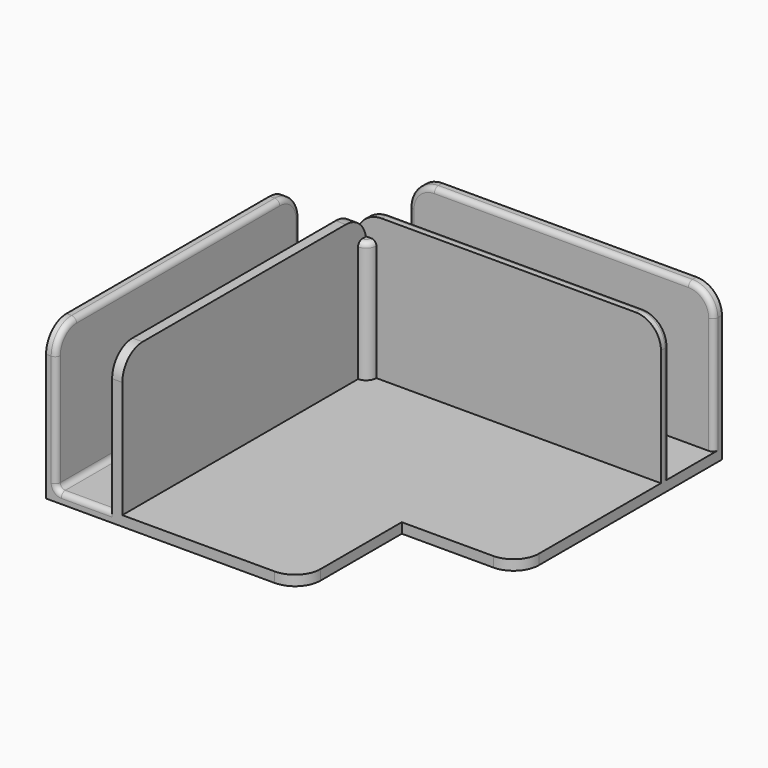
from build123d import *

# Parameters (mm, degrees)
F0_W         = 2
F0_H         = 2
F0_W_2       = 11
F0_H_2       = 28
F0_W_3       = 35
F1_DEPTH     = 60
F2_ANGLE     = -90
F4_R         = 5
F4_2_R       = 5
F6_DEPTH     = 23.9
F7_R         = 1.99999
F8_T1_DEPTH  = 60
F8_T3_DEPTH  = 23
F8_T5_DEPTH  = 1e-05
F8_T7_DEPTH  = 1e-05
F8_T9_DEPTH  = 50
F8_T12_ANGLE = 90
F8_T14_ANGLE = 90
F8_T16_ANGLE = 90
F8_T18_ANGLE = 90
F8_T20_ANGLE = 90
F8_T21_DEPTH = 50
F8_T23_DEPTH = 22
F8_T25_DEPTH = 10
F8_T28_ANGLE = 90
F8_T30_ANGLE = 90
F8_T32_ANGLE = 90
F8_T34_ANGLE = 90


# Not quite as in the source:
# - a fillet or chamfer that OpenCascade refuses, or shapes differently, is made with other operations: its cross-section is extruded or revolved along the edge and cut away or added
# - a fillet or chamfer is up to 0.001 mm smaller than in the source, because OpenCascade refuses the exact size


with BuildPart() as f1:
    # F0 (on Front) → F1 (new body)
    with BuildSketch(Plane.XZ):
        with Locations((1, 1)):
            Rectangle(F0_W, F0_H)
        with Locations((7.5, 1)):
            Rectangle(F0_W_2, F0_H)
        with Locations((1, 16)):
            Rectangle(F0_W, F0_H_2)
        with Locations((14, 1)):
            Rectangle(F0_W, F0_H)
        with Locations((32.5, 1)):
            Rectangle(F0_W_3, F0_H)
        with Locations((14, 16)):
            Rectangle(F0_W, F0_H_2)
    extrude(amount=F1_DEPTH)


with BuildPart() as f2_1:
    # F2: copy of F1
    add(f1.part.rotate(Axis((15, 0, 16), (0, 0, 1)), F2_ANGLE))


with BuildPart() as f2_1_1:
    # F3: moved
    add(f2_1.part.moved(Location((58, 0, 0))))

    # F4#2
    f4_2_edges = [f2_1_1.edges().sort_by_distance(p)[0] for p in [
        (73, 1, 30),
        (73, 14, 30),
        (13, 14, 30),
        (13, 1, 30),
        (73, -35, 1),
    ]]
    fillet(f4_2_edges, radius=F4_2_R)


with BuildPart() as f1_1:
    add(f1.part)

    # F4
    f4_edges = [f1_1.edges().sort_by_distance(p)[0] for p in [
        (14, 0, 30),
        (1, 0, 30),
        (14, -60, 30),
        (1, -60, 30),
        (50, -60, 1),
    ]]
    fillet(f4_edges, radius=F4_R)

    add(f2_1_1.part)  # F6 merges F2_1
    # F5 (on face) → F6 (join)
    with BuildSketch(Plane.XY.offset(2)):
        Polygon((16.8020091951, 0), (15, 0), (15, -2), (17, -2), (17, 0), align=None)
    extrude(amount=F6_DEPTH)

    # F7 (radius 2 in the source; OpenCascade refuses exactly that, so slightly less here)
    f7_edges = [f1_1.edges().sort_by_distance(p)[0] for p in [
        (17, -2, 13.95),
    ]]
    fillet(f7_edges, radius=F7_R)

    # F8: fillet of radius 1 on 19 edges, made by hand

    # F8_s2 → F8_t1 (join)
    with BuildSketch(Plane.XZ):
        with BuildLine():
            ThreePointArc((2, 3), (2.2928932188, 2.2928932188), (3, 2))
            Line((3, 2), (2, 2))
            Line((2, 2), (2, 3))
        make_face()
    extrude(amount=F8_T1_DEPTH)

    # F8_s4 → F8_t3 (cut)
    with BuildSketch(Plane.XY.offset(2)):
        with BuildLine():
            ThreePointArc((13, 1), (13.2928932188, 1.7071067812), (14, 2))
            Line((14, 2), (13, 2))
            Line((13, 2), (13, 1))
        make_face()
        with BuildLine():
            ThreePointArc((73, 14), (72.7071067812, 13.2928932188), (72, 13))
            Line((72, 13), (73, 13))
            Line((73, 13), (73, 14))
        make_face()
        with BuildLine():
            ThreePointArc((73, 1), (72.7071067812, 1.7071067812), (72, 2))
            Line((72, 2), (73, 2))
            Line((73, 2), (73, 1))
        make_face()
        with BuildLine():
            ThreePointArc((13, 14), (13.2928932188, 13.2928932188), (14, 13))
            Line((14, 13), (13, 13))
            Line((13, 13), (13, 14))
        make_face()
    extrude(amount=F8_T3_DEPTH, mode=Mode.SUBTRACT)

    # F8_s6 → F8_t5 (cut)
    with BuildSketch(Plane.YZ.offset(15)):
        with BuildLine():
            ThreePointArc((-2, 24.9), (-1.7071067812, 25.6071067812), (-1, 25.9))
            Line((-1, 25.9), (-2, 25.9))
            Line((-2, 25.9), (-2, 24.9))
        make_face()
    extrude(amount=F8_T5_DEPTH, mode=Mode.SUBTRACT)

    # F8_s8 → F8_t7 (cut)
    with BuildSketch(Plane.XZ):
        with BuildLine():
            ThreePointArc((17, 24.9), (16.7071067812, 25.6071067812), (16, 25.9))
            Line((16, 25.9), (17, 25.9))
            Line((17, 25.9), (17, 24.9))
        make_face()
    extrude(amount=F8_T7_DEPTH, mode=Mode.SUBTRACT)

    # F8_s10 → F8_t9 (cut)
    with BuildSketch(Plane.YZ.offset(18)):
        with BuildLine():
            ThreePointArc((13, 29), (13.2928932188, 29.7071067812), (14, 30))
            Line((14, 30), (13, 30))
            Line((13, 30), (13, 29))
        make_face()
        with BuildLine():
            ThreePointArc((1, 30), (1.7071067812, 29.7071067812), (2, 29))
            Line((2, 29), (2, 30))
            Line((2, 30), (1, 30))
        make_face()
    extrude(amount=F8_T9_DEPTH, mode=Mode.SUBTRACT)

    # F8_s11 → F8_t12 (revolve, cut)
    with BuildSketch(Plane.XZ.offset(1e-05)):
        with BuildLine():
            ThreePointArc((17, 24.9), (16.7071067812, 25.6071067812), (16, 25.9))
            Line((16, 25.9), (17, 25.9))
            Line((17, 25.9), (17, 24.9))
        make_face()
    revolve(axis=Axis((15.00001, -1e-05, 25.9), (0, 0, -1)), revolution_arc=F8_T12_ANGLE, mode=Mode.SUBTRACT)

    # F8_s13 → F8_t14 (revolve, cut)
    with BuildSketch(Plane.YZ.offset(68)):
        with BuildLine():
            ThreePointArc((1, 30), (1.7071067812, 29.7071067812), (2, 29))
            Line((2, 29), (2, 30))
            Line((2, 30), (1, 30))
        make_face()
    revolve(axis=Axis((68, 2, 25), (0, 1, 0)), revolution_arc=F8_T14_ANGLE, mode=Mode.SUBTRACT)

    # F8_s15 → F8_t16 (revolve, cut)
    with BuildSketch(Plane.YZ.offset(18)):
        with BuildLine():
            ThreePointArc((1, 30), (1.7071067812, 29.7071067812), (2, 29))
            Line((2, 29), (2, 30))
            Line((2, 30), (1, 30))
        make_face()
    revolve(axis=Axis((18, 2, 25), (0, -1, 0)), revolution_arc=F8_T16_ANGLE, mode=Mode.SUBTRACT)

    # F8_s17 → F8_t18 (revolve, cut)
    with BuildSketch(Plane.YZ.offset(68)):
        with BuildLine():
            ThreePointArc((14, 30), (13.2928932188, 29.7071067812), (13, 29))
            Line((13, 29), (13, 30))
            Line((13, 30), (14, 30))
        make_face()
    revolve(axis=Axis((68, 13, 25), (0, 1, 0)), revolution_arc=F8_T18_ANGLE, mode=Mode.SUBTRACT)

    # F8_s19 → F8_t20 (revolve, cut)
    with BuildSketch(Plane.YZ.offset(18)):
        with BuildLine():
            ThreePointArc((13, 29), (13.2928932188, 29.7071067812), (14, 30))
            Line((14, 30), (13, 30))
            Line((13, 30), (13, 29))
        make_face()
    revolve(axis=Axis((18, 13, 25), (0, -1, 0)), revolution_arc=F8_T20_ANGLE, mode=Mode.SUBTRACT)

    # F8_s22 → F8_t21 (cut)
    with BuildSketch(Plane.XZ.offset(5)):
        with BuildLine():
            ThreePointArc((2, 29), (1.7071067812, 29.7071067812), (1, 30))
            Line((1, 30), (2, 30))
            Line((2, 30), (2, 29))
        make_face()
    extrude(amount=F8_T21_DEPTH, mode=Mode.SUBTRACT)

    # F8_s24 → F8_t23 (cut)
    with BuildSketch(Plane.XY.offset(3)):
        with BuildLine():
            ThreePointArc((2, -1), (1.7071067812, -0.2928932188), (1, 0))
            Line((1, 0), (2, 0))
            Line((2, 0), (2, -1))
        make_face()
        with BuildLine():
            ThreePointArc((2, -59), (1.7071067812, -59.7071067812), (1, -60))
            Line((1, -60), (2, -60))
            Line((2, -60), (2, -59))
        make_face()
    extrude(amount=F8_T23_DEPTH, mode=Mode.SUBTRACT)

    # F8_s26 → F8_t25 (cut)
    with BuildSketch(Plane.YZ.offset(3)):
        with BuildLine():
            ThreePointArc((-59, 2), (-59.7071067812, 1.7071067812), (-60, 1))
            Line((-60, 1), (-60, 2))
            Line((-60, 2), (-59, 2))
        make_face()
        with BuildLine():
            ThreePointArc((-1, 2), (-0.2928932188, 1.7071067812), (0, 1))
            Line((0, 1), (0, 2))
            Line((0, 2), (-1, 2))
        make_face()
    extrude(amount=F8_T25_DEPTH, mode=Mode.SUBTRACT)

    # F8_s27 → F8_t28 (revolve, cut)
    with BuildSketch(Plane.XZ.offset(5)):
        with BuildLine():
            ThreePointArc((2, 29), (1.7071067812, 29.7071067812), (1, 30))
            Line((1, 30), (2, 30))
            Line((2, 30), (2, 29))
        make_face()
    revolve(axis=Axis((2, -5, 25), (-1, 0, 0)), revolution_arc=F8_T28_ANGLE, mode=Mode.SUBTRACT)

    # F8_s29 → F8_t30 (revolve, cut)
    with BuildSketch(Plane.XZ.offset(55)):
        with BuildLine():
            ThreePointArc((1, 30), (1.7071067812, 29.7071067812), (2, 29))
            Line((2, 29), (2, 30))
            Line((2, 30), (1, 30))
        make_face()
    revolve(axis=Axis((2, -55, 25), (1, 0, 0)), revolution_arc=F8_T30_ANGLE, mode=Mode.SUBTRACT)

    # F8_s31 → F8_t32 (revolve, cut)
    with BuildSketch(Plane.XY.offset(3)):
        with BuildLine():
            ThreePointArc((2, -1), (1.7071067812, -0.2928932188), (1, 0))
            Line((1, 0), (2, 0))
            Line((2, 0), (2, -1))
        make_face()
    revolve(axis=Axis((3, 0, 3), (0, -1, 0)), revolution_arc=F8_T32_ANGLE, mode=Mode.SUBTRACT)

    # F8_s33 → F8_t34 (revolve, cut)
    with BuildSketch(Plane.XY.offset(3)):
        with BuildLine():
            ThreePointArc((2, -59), (1.7071067812, -59.7071067812), (1, -60))
            Line((1, -60), (2, -60))
            Line((2, -60), (2, -59))
        make_face()
    revolve(axis=Axis((3, -60, 3), (0, -1, 0)), revolution_arc=F8_T34_ANGLE, mode=Mode.SUBTRACT)


solid = f1_1.part
